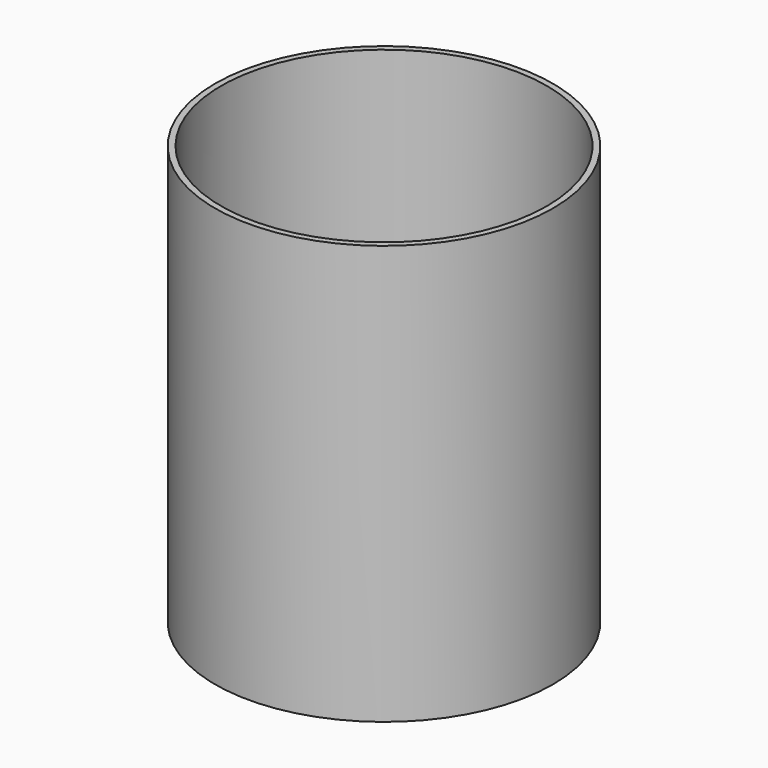
from build123d import *

# Parameters (mm, degrees)
F2_R     = 34.75
F2_R_2   = 33.5
F3_DEPTH = 86.2


with BuildPart() as f3:
    # F2 (on Top) → F3 (new body)
    with BuildSketch(Plane.XY):
        Circle(F2_R)
        Circle(F2_R_2, mode=Mode.SUBTRACT)
    extrude(amount=F3_DEPTH)


solid = f3.part
